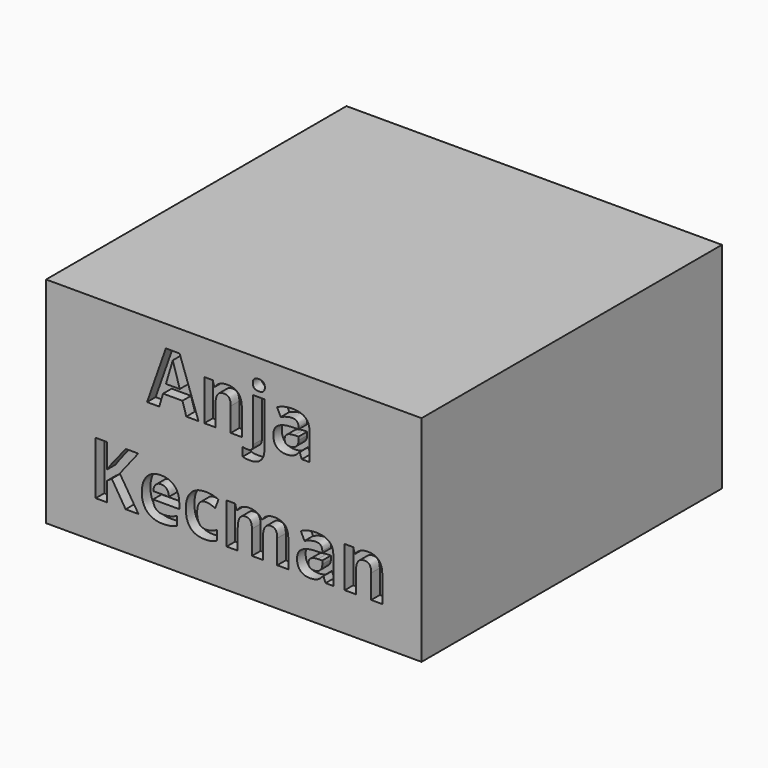
from build123d import *

# Parameters (mm, degrees)
F0_W         = 35
F0_H         = 35
F1_DEPTH     = 20
F2_TEXT_SIZE = 6.9444444444
F3_DEPTH     = 1


# Not quite as in the source:
# - Text() gives the source's letters only with a copy of the font that has no kerning and outlines rounded to 1/6400 em; it was checked with that copy


with BuildPart() as f1:
    # F0 (on Top) → F1 (new body)
    with BuildSketch(Plane.XY):
        with Locations((17.5, 17.5)):
            Rectangle(F0_W, F0_H)
    extrude(amount=F1_DEPTH)

    # F2 (on face) → F3 (cut)
    with BuildSketch(Plane.XZ):
        with Locations((9.4134114583, 13)):
            Text('Anja', F2_TEXT_SIZE, font='Open Sans', font_style=FontStyle.BOLD, text_align=(TextAlign.LEFT, TextAlign.BOTTOM))
        with Locations((4, 3.5555555556)):
            Text('Kecman', F2_TEXT_SIZE, font='Open Sans', font_style=FontStyle.BOLD, text_align=(TextAlign.LEFT, TextAlign.BOTTOM))
    extrude(amount=-F3_DEPTH, mode=Mode.SUBTRACT)


solid = f1.part
